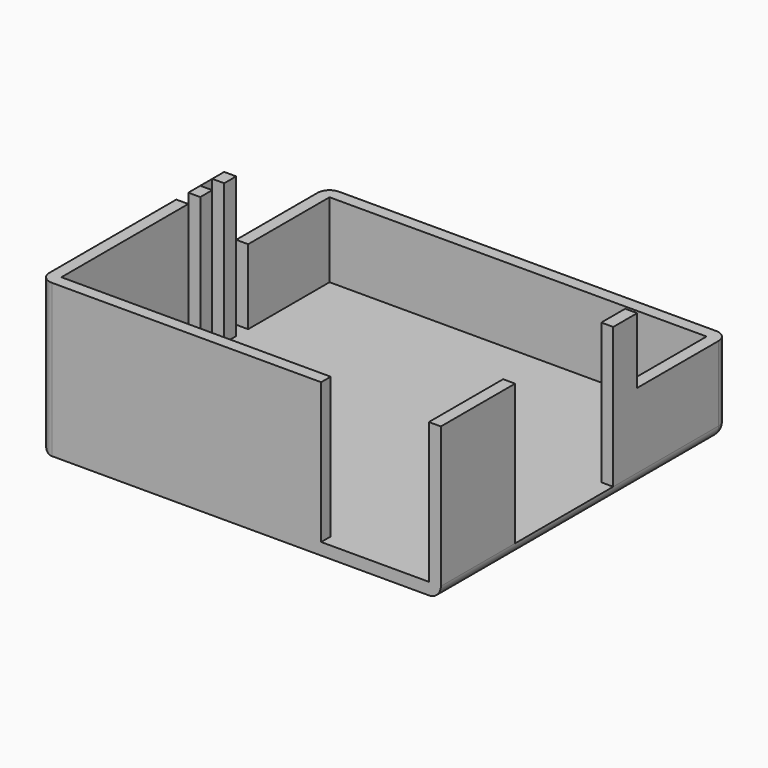
from build123d import *

# Parameters (mm, degrees)
F0_W     = 4
F0_H     = 41
F0_H_2   = 10
F0_H_3   = 5
F0_W_2   = 36
F0_H_4   = 4
F0_W_3   = 126
F0_H_5   = 34
F1_DEPTH = 4
F2_DEPTH = 51
F3_DEPTH = 29
F4_R     = 3.99999
F5_DEPTH = 51
F6_R     = 3.99999


# Not quite as in the source:
# - a fillet or chamfer is up to 0.001 mm smaller than in the source, because OpenCascade refuses the exact size
# - a feature names something its author has since deleted; it is built from what else it names


with BuildPart() as f1:
    # F0 (on Top) → F1 (new body)
    with BuildSketch(Plane.XY):
        Polygon((36, 82), (40, 82), (40, 120), (-94, 120), (-94, 82), (-90, 82), (-90, 116), (36, 116), align=None)
        Polygon((-94, 0), (0, 0), (0, 4), (-90, 4), (-90, 57), (-94, 57), align=None)
        with Locations((38, 51.5)):
            Rectangle(F0_W, F0_H)
        with Locations((38, 77)):
            Rectangle(F0_W, F0_H_2)
        with Locations((-92, 79.5)):
            Rectangle(F0_W, F0_H_3)
        with Locations((-92, 59.5)):
            Rectangle(F0_W, F0_H_3)
        with Locations((-92, 69.5)):
            Rectangle(F0_W, F0_H_3)
        with Locations((-92, 74.5)):
            Rectangle(F0_W, F0_H_3)
        with Locations((-92, 64.5)):
            Rectangle(F0_W, F0_H_3)
        with Locations((18, 2)):
            Rectangle(F0_W_2, F0_H_4)
        with Locations((-27, 99)):
            Rectangle(F0_W_3, F0_H_5)
        Polygon((-90, 4), (0, 4), (36, 4), (36, 31), (36, 72), (36, 82), (-90, 82), (-90, 77), (-90, 72), (-90, 67), (-90, 62), (-90, 57), align=None)
    extrude(amount=F1_DEPTH)

    # F0 (on Top) → F2 (join)
    with BuildSketch(Plane.XY):
        Polygon((36, 4), (36, 0), (40, 0), (40, 31), (36, 31), align=None)
        with Locations((38, 77)):
            Rectangle(F0_W, F0_H_2)
        Polygon((-94, 0), (0, 0), (0, 4), (-90, 4), (-90, 57), (-94, 57), align=None)
    extrude(amount=F2_DEPTH)

    # F0 (on Top) → F3 (join)
    with BuildSketch(Plane.XY):
        Polygon((36, 82), (40, 82), (40, 120), (-94, 120), (-94, 82), (-90, 82), (-90, 116), (36, 116), align=None)
    extrude(amount=F3_DEPTH)

    # F4 (radius 4 in the source; OpenCascade refuses exactly that, so slightly less here)
    f4_edges = [f1.edges().sort_by_distance(p)[0] for p in [
        (40, 60, 0),
        (-27, 120, 0),
        (40, 120, 14.5),
        (-94, 120, 14.5),
        (-94, 60, 0),
        (-94, 0, 25.5),
    ]]
    fillet(f4_edges, radius=F4_R)

    # F0 (on Top) → F5 (join)
    with BuildSketch(Plane.XY):
        with Locations((-92, 74.5)):
            Rectangle(F0_W, F0_H_3)
        with Locations((-92, 64.5)):
            Rectangle(F0_W, F0_H_3)
    extrude(amount=F5_DEPTH)

    # F6 (radius 4 in the source; OpenCascade refuses exactly that, so slightly less here)
    f6_edges = [f1.edges().sort_by_distance(p)[0] for p in [
        (-94, 74.5, 0),
        (-94, 64.5, 0),
    ]]
    fillet(f6_edges, radius=F6_R)


solid = f1.part
